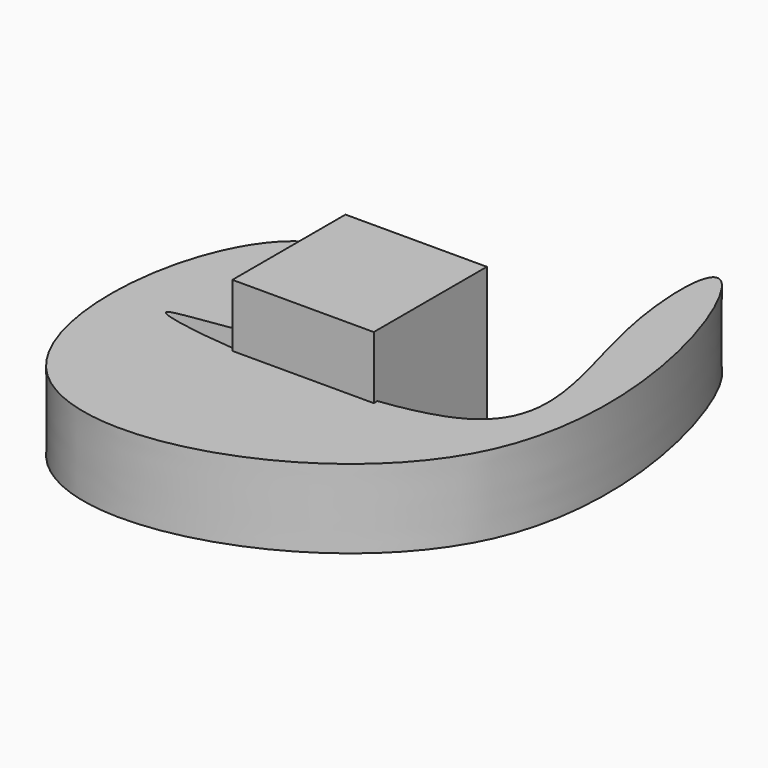
from build123d import *

# Parameters (mm, degrees)
F0_W     = 50
F0_H     = 50
F1_DEPTH = 50
F3_DEPTH = 27.8581473976


# Not quite as in the source:
# - a feature names something its author has since deleted; it is built from what else it names


with BuildPart() as f1:
    # F0 (on Top) → F1 (new body)
    with BuildSketch(Plane.XY):
        Rectangle(F0_W, F0_H)
    extrude(amount=F1_DEPTH)

    # F2 (on Top) → F3 (join)
    with BuildSketch(Plane.XY):
        with BuildLine():
            add(Edge.make_bspline(
                [(52.3223727942, 52.3223653436), (58.4426768344, 24.6124569356), (89.0864693147, -39.0035553174), (-113.7436141158, -15.5521322754), (38.4040637994, -14.655780005), (-64.7631097157, 87.9831313006), (-96.0872297903, -118.0362663459), (116.6700963492, -52.8790603504), (47.0078253263, 130.2848007445), (47.6236481067, 73.5960193758), (52.3223727942, 52.3223653436)],
                knots=[0, 0, 0, 0, 0.1134180678, 0.2535365417, 0.3567310586, 0.4632609861, 0.6058085851, 0.7630573143, 0.9129258495, 1, 1, 1, 1], degree=3))
        make_face()
    extrude(amount=F3_DEPTH)


solid = f1.part
